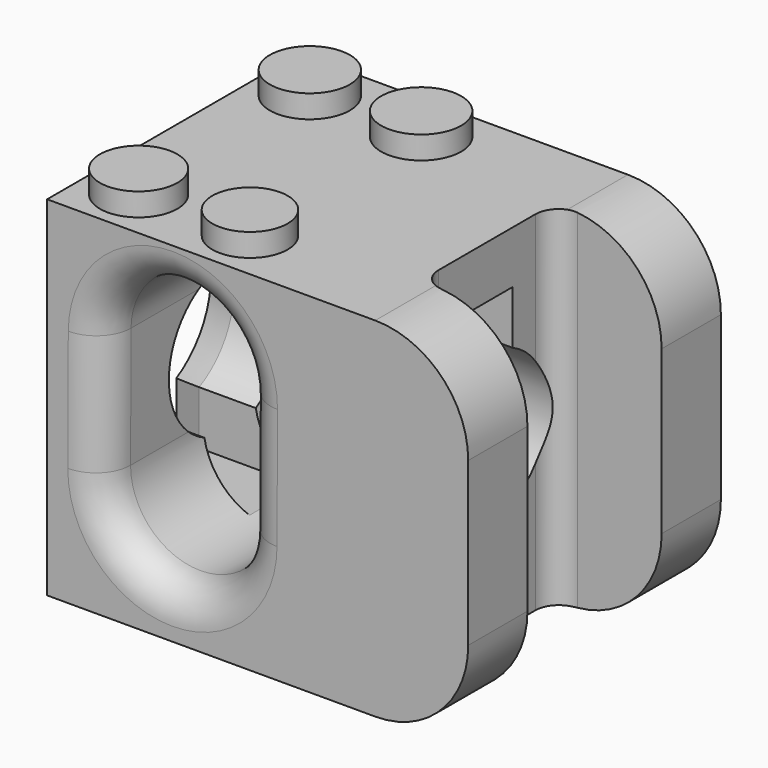
from build123d import *

# Parameters (mm, degrees)
F1_DEPTH               = 76.2
F2_R                   = 20.32
F3_R                   = 5.08
F5_DEPTH               = 69.0143647131
F6_R                   = 7.62
F8_DEPTH               = 92.0188220676
F9_DEPTH               = 6.35
DRAFT_F9_DRAFTED_ANGLE = 15
F10_R                  = 8.7391838485
F10_R_2                = 8.7468633962
F10_R_3                = 8.4686200881
F10_R_4                = 8.240890104
F11_DEPTH              = 5


# Not quite as in the source:
# - an extrude with a draft is written as a straight extrude whose walls are then drafted


with BuildPart() as f1:
    # F0 (on Top) → F1 (new body)
    with BuildSketch(Plane.XY):
        Polygon((13.9037920162, 0), (-54.6039827168, 0), (-54.6039827168, -34.5066823065), (37.4138392508, -34.5066823065), (37.4138392508, -18.3277260512), (13.9037920162, -18.3277260512), align=None)
        Polygon((37.4138392508, 34.5066823065), (-54.6039827168, 34.5066823065), (-54.6039827168, 0), (13.9037920162, 0), (13.9037920162, 18.3277260512), (37.4138392508, 18.3277260512), align=None)
    extrude(amount=F1_DEPTH)

    # F2
    f2_edges = [f1.edges().sort_by_distance(p)[0] for p in [
        (37.413839, -26.417204, 76.2),
        (37.413839, 26.417204, 76.2),
        (37.413839, 26.417204, 0),
        (37.413839, -26.417204, 0),
    ]]
    fillet(f2_edges, radius=F2_R)

    # F3
    f3_edges = [f1.edges().sort_by_distance(p)[0] for p in [
        (13.903792, 18.327726, 38.1),
        (13.903792, -18.327726, 38.1),
    ]]
    fillet(f3_edges, radius=F3_R)

    # F4 (on face) → F5 (cut, through all)
    with BuildSketch(Plane.XZ.offset(34.5066823065)):
        with BuildLine():
            Line((-42.3591247506, 52.2906772566), (-42.4619570783, 25.878727725))
            ThreePointArc((-42.4619570783, 25.878727725), (-27.2814075766, 10.5795082408), (-11.9821880924, 25.7600577424))
            Line((-11.9821880924, 25.7600577424), (-11.8793557647, 52.172007274))
            ThreePointArc((-11.8793557647, 52.172007274), (-27.0599052664, 67.4712267583), (-42.3591247506, 52.2906772566))
        make_face()
    extrude(amount=-F5_DEPTH, mode=Mode.SUBTRACT)

    # F6
    f6_edges = [f1.edges().sort_by_distance(p)[0] for p in [
        (-27.059905, -34.506682, 67.471227),
        (-42.359125, 0, 52.290677),
        (-27.059905, 34.506682, 67.471227),
        (-11.879356, 0, 52.172007),
        (-27.281408, -34.506682, 10.579508),
        (-42.410541, -34.506682, 39.084702),
        (-11.930772, -34.506682, 38.966033),
        (-11.930772, 34.506682, 38.966033),
        (-42.410541, 34.506682, 39.084702),
        (-27.281408, 34.506682, 10.579508),
    ]]
    fillet(f6_edges, radius=F6_R)

    # F7 (on face) → F8 (cut, through all)
    with BuildSketch(Plane(origin=(-54.6039827168, 0, 0), x_dir=(0, -1, 0), z_dir=(-1, 0, 0))):
        with BuildLine():
            Line((7.0178462192, 11.4734675735), (7.0178462192, 23.1743131117))
            ThreePointArc((7.0178462192, 23.1743131117), (16.4932196567, 38.1), (7.0178462192, 53.0256868883))
            Line((7.0178462192, 53.0256868883), (7.0178462192, 64.7265324265))
            Line((7.0178462192, 64.7265324265), (-7.0178462192, 64.7265324265))
            Line((-7.0178462192, 64.7265324265), (-7.0178462192, 53.0256868883))
            ThreePointArc((-7.0178462192, 53.0256868883), (-16.4932196567, 38.1), (-7.0178462192, 23.1743131117))
            Line((-7.0178462192, 23.1743131117), (-7.0178462192, 11.4734675735))
            Line((-7.0178462192, 11.4734675735), (7.0178462192, 11.4734675735))
        make_face()
    extrude(amount=-F8_DEPTH, mode=Mode.SUBTRACT)


with BuildPart() as f9_drafted:
    # F7 (on face) → F9 (new body)
    with BuildSketch(Plane(origin=(-54.6039827168, 0, 0), x_dir=(0, -1, 0), z_dir=(-1, 0, 0))):
        with BuildLine():
            Line((-13.3678462192, 71.0765324265), (-13.3678462192, 56.6233196739))
            ThreePointArc((-13.3678462192, 56.6233196739), (-22.8432196567, 38.1), (-13.3678462192, 19.5766803261))
            Line((-13.3678462192, 19.5766803261), (-13.3678462192, 5.1234675735))
            Line((-13.3678462192, 5.1234675735), (13.3678462192, 5.1234675735))
            Line((13.3678462192, 5.1234675735), (13.3678462192, 19.5766803261))
            ThreePointArc((13.3678462192, 19.5766803261), (22.8432196567, 38.1), (13.3678462192, 56.6233196739))
            Line((13.3678462192, 56.6233196739), (13.3678462192, 71.0765324265))
            Line((13.3678462192, 71.0765324265), (-13.3678462192, 71.0765324265))
        make_face()
        with BuildLine():
            ThreePointArc((7.0178462192, 53.0256868883), (16.4932196567, 38.1), (7.0178462192, 23.1743131117))
            Line((7.0178462192, 23.1743131117), (7.0178462192, 11.4734675735))
            Line((7.0178462192, 11.4734675735), (-7.0178462192, 11.4734675735))
            Line((-7.0178462192, 11.4734675735), (-7.0178462192, 23.1743131117))
            ThreePointArc((-7.0178462192, 23.1743131117), (-16.4932196567, 38.1), (-7.0178462192, 53.0256868883))
            Line((-7.0178462192, 53.0256868883), (-7.0178462192, 64.7265324265))
            Line((-7.0178462192, 64.7265324265), (7.0178462192, 64.7265324265))
            Line((7.0178462192, 64.7265324265), (7.0178462192, 53.0256868883))
        make_face(mode=Mode.SUBTRACT)
    extrude(amount=F9_DEPTH)

    # draft_F9_drafted
    draft_f9_drafted_walls = [f9_drafted.faces().sort_by_distance(p)[0] for p in [
        (-58.8373160501, -13.3678462192, 63.8499260502),
        (-58.8373160501, 0, 71.0765324265),
        (-58.8373160501, 13.3678462192, 63.8499260502),
        (-58.8373160501, 22.8432196567, 38.1),
        (-58.8373160501, 13.3678462192, 12.3500739498),
        (-58.8373160501, 0, 5.1234675735),
        (-58.8373160501, -13.3678462192, 12.3500739498),
        (-58.8373160501, -22.8432196567, 38.1),
        (-58.8373160501, -16.4932196567, 38.1),
        (-58.8373160501, -7.0178462192, 17.3238903426),
        (-58.8373160501, 0, 11.4734675735),
        (-58.8373160501, 7.0178462192, 17.3238903426),
        (-58.8373160501, 16.4932196567, 38.1),
        (-58.8373160501, 7.0178462192, 58.8761096574),
        (-58.8373160501, 0, 64.7265324265),
        (-58.8373160501, -7.0178462192, 58.8761096574),
    ]]
    draft(draft_f9_drafted_walls, neutral_plane=Plane(origin=(-54.6039827168, 0, 0), x_dir=(0, -1, 0), z_dir=(-1, 0, 0)), angle=DRAFT_F9_DRAFTED_ANGLE)


with BuildPart() as f1_1:
    add(f1.part)

    # join_F9_drafted: union F9_drafted
    add(f9_drafted.part)

    # F10 (on face) → F11 (join)
    with BuildSketch(Plane.XY.offset(76.2)):
        with Locations((-43.5103178024, 23.3799535781)):
            Circle(F10_R)
        with Locations((-19.1782396287, 23.3799535781)):
            Circle(F10_R_2)
        with Locations((-43.5103178024, -23.3799610287)):
            Circle(F10_R_3)
        with Locations((-19.1782396287, -23.3799610287)):
            Circle(F10_R_4)
    extrude(amount=F11_DEPTH)


solid = f1_1.part
